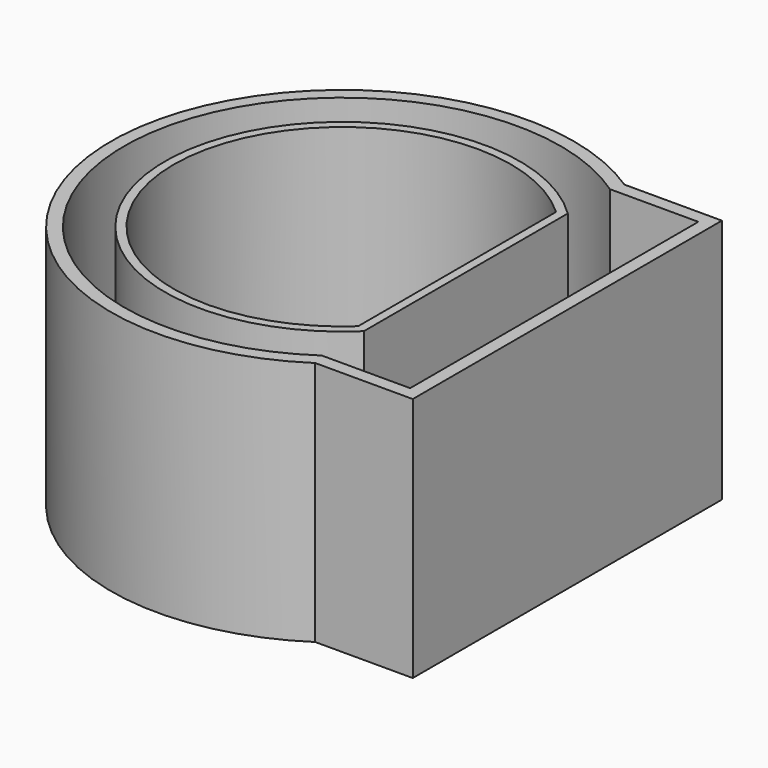
from build123d import *

# Parameters (mm, degrees)
F1_DEPTH = 1.5
F2_DEPTH = 22.5
F4_DEPTH = 25


# Not quite as in the source:
# - a feature names something its author has since deleted; it is built from what else it names


with BuildPart() as f1:
    # F0 (on Top) → F1 (new body)
    with BuildSketch(Plane.XY):
        with BuildLine():
            Line((20.6026545555, 17.7), (11.6683332143, 17.7))
            ThreePointArc((11.6683332143, 17.7), (-21.2, 0), (11.6683332143, -17.7))
            Line((11.6683332143, -17.7), (20.6026545555, -17.7))
            Line((20.6026545555, -17.7), (20.6026545555, 17.7))
        make_face()
        with BuildLine():
            ThreePointArc((11.3026545555, -16.5), (-20, 0), (11.3026545555, 16.5))
            Line((11.3026545555, 16.5), (19.4026545555, 16.5))
            Line((19.4026545555, 16.5), (19.4026545555, -16.5))
            Line((19.4026545555, -16.5), (11.3026545555, -16.5))
        make_face(mode=Mode.SUBTRACT)
        with BuildLine():
            Line((19.4026545555, 16.5), (11.3026545555, 16.5))
            ThreePointArc((11.3026545555, 16.5), (-20, 0), (11.3026545555, -16.5))
            Line((11.3026545555, -16.5), (19.4026545555, -16.5))
            Line((19.4026545555, -16.5), (19.4026545555, 16.5))
        make_face()
        with BuildLine():
            ThreePointArc((11.3026545555, -11.6752944288), (-16.25, 0), (11.3026545555, 11.6752944288))
            Line((11.3026545555, 11.6752944288), (11.3026545555, -11.6752944288))
        make_face(mode=Mode.SUBTRACT)
        with BuildLine():
            Line((11.3026545555, -11.6752944288), (11.3026545555, 11.6752944288))
            ThreePointArc((11.3026545555, 11.6752944288), (-16.25, 0), (11.3026545555, -11.6752944288))
        make_face()
        with BuildLine():
            ThreePointArc((10.5026545555, -11.3312288517), (-15.45, 0), (10.5026545555, 11.3312288517))
            Line((10.5026545555, 11.3312288517), (10.5026545555, -11.3312288517))
        make_face(mode=Mode.SUBTRACT)
        with BuildLine():
            Line((10.5026545555, -11.3312288517), (10.5026545555, 11.3312288517))
            ThreePointArc((10.5026545555, 11.3312288517), (-15.45, 0), (10.5026545555, -11.3312288517))
        make_face()
    extrude(amount=F1_DEPTH)

    # F0 (on Top) → F2 (join)
    with BuildSketch(Plane.XY):
        with BuildLine():
            Line((20.6026545555, 17.7), (11.6683332143, 17.7))
            ThreePointArc((11.6683332143, 17.7), (-21.2, 0), (11.6683332143, -17.7))
            Line((11.6683332143, -17.7), (20.6026545555, -17.7))
            Line((20.6026545555, -17.7), (20.6026545555, 17.7))
        make_face()
        with BuildLine():
            ThreePointArc((11.3026545555, -16.5), (-20, 0), (11.3026545555, 16.5))
            Line((11.3026545555, 16.5), (19.4026545555, 16.5))
            Line((19.4026545555, 16.5), (19.4026545555, -16.5))
            Line((19.4026545555, -16.5), (11.3026545555, -16.5))
        make_face(mode=Mode.SUBTRACT)
        with BuildLine():
            Line((11.3026545555, -11.6752944288), (11.3026545555, 11.6752944288))
            ThreePointArc((11.3026545555, 11.6752944288), (-16.25, 0), (11.3026545555, -11.6752944288))
        make_face()
        with BuildLine():
            ThreePointArc((10.5026545555, -11.3312288517), (-15.45, 0), (10.5026545555, 11.3312288517))
            Line((10.5026545555, 11.3312288517), (10.5026545555, -11.3312288517))
        make_face(mode=Mode.SUBTRACT)
    extrude(amount=F2_DEPTH)

    # F3 (on face) → F4 (cut)
    with BuildSketch(Plane.XY.offset(1.5)):
        Polygon((19.4026545555, 16.5), (11.3026545555, 16.5), (11.3026545555, 11.6752944288), (11.3026545555, -11.6752944288), (11.3026545555, -16.5), (19.4026545555, -16.5), align=None)
    extrude(amount=-F4_DEPTH, mode=Mode.SUBTRACT)


solid = f1.part
